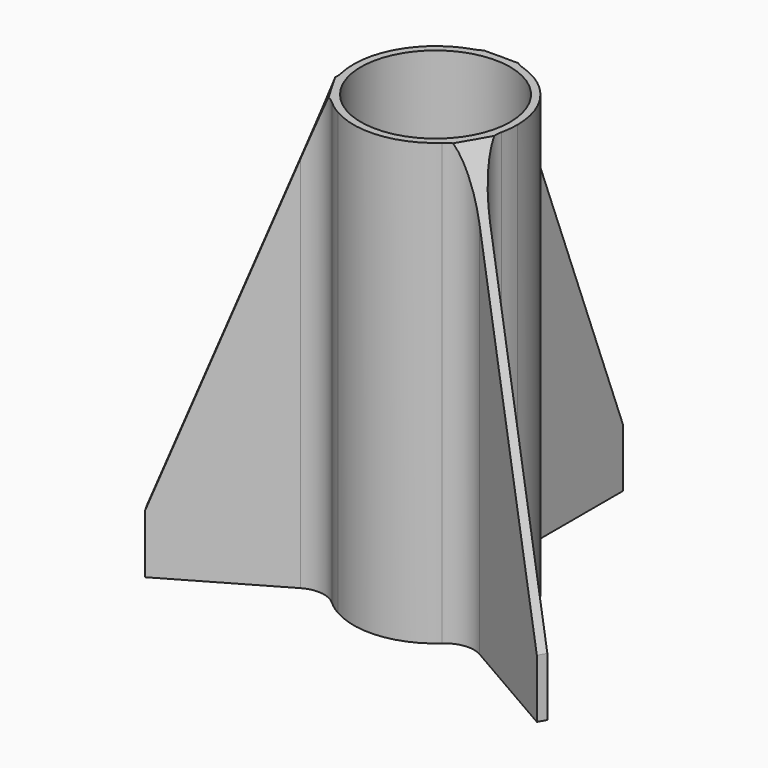
from build123d import *

# Parameters (mm, degrees)
F0_R     = 12.7
F1_DEPTH = 75
F3_DEPTH = 1.5
F4_R     = 5
F6_COUNT = 3
F6_ANGLE = 240


# Not quite as in the source:
# - a feature names something its author has since deleted; it is built from what else it names


with BuildPart() as f1:
    # F0 (on Top) → F1 (new body)
    with BuildSketch(Plane.XY):
        with BuildLine():
            ThreePointArc((-0.75, 13.9298241195), (-9.595311355, -10.125833299), (13.95, 0))
            ThreePointArc((13.95, 0), (10.125833299, 9.595311355), (0.75, 13.9298241195))
            ThreePointArc((0.75, 13.9298241195), (0, 13.95), (-0.75, 13.9298241195))
        make_face()
        Circle(F0_R, mode=Mode.SUBTRACT)
        with BuildLine():
            ThreePointArc((-0.75, 13.9298241195), (0, 13.95), (0.75, 13.9298241195))
            Line((0.75, 13.9298241195), (0.75, 38.9298241195))
            Line((0.75, 38.9298241195), (0, 38.9298241195))
            Line((0, 38.9298241195), (-0.75, 38.9298241195))
            Line((-0.75, 38.9298241195), (-0.75, 13.9298241195))
        make_face()
    extrude(amount=F1_DEPTH)

    # F2 (on face) → F3 (cut, through all)
    with BuildSketch(Plane.YZ.offset(0.75)):
        Polygon((38.9298241195, 75), (13.9298241195, 75), (38.9298241195, 10), align=None)
    extrude(amount=-F3_DEPTH, mode=Mode.SUBTRACT)

    # F4 (call 1 of 2: OpenCascade refuses the feature's edges together)
    f4_edges = [f1.edges().sort_by_distance(p)[0] for p in [
        (0.75, 13.929824, 37.5),
    ]]
    fillet(f4_edges, radius=F4_R)

    # F4#2 (call 2 of 2)
    f4_2_edges = [f1.edges().sort_by_distance(p)[0] for p in [
        (-0.75, 13.929824, 37.5),
    ]]
    fillet(f4_2_edges, radius=F4_R)

    # F6: F1 ×3 about axis
    f6_axis = Axis((0, 0, 42.7156351507), (0, 0, 1))


with BuildPart() as f1_1:
    add(f1.part)
    for i in range(1, F6_COUNT):
        add(f1.part.rotate(f6_axis, i * F6_ANGLE / (F6_COUNT - 1)))


solid = f1_1.part
